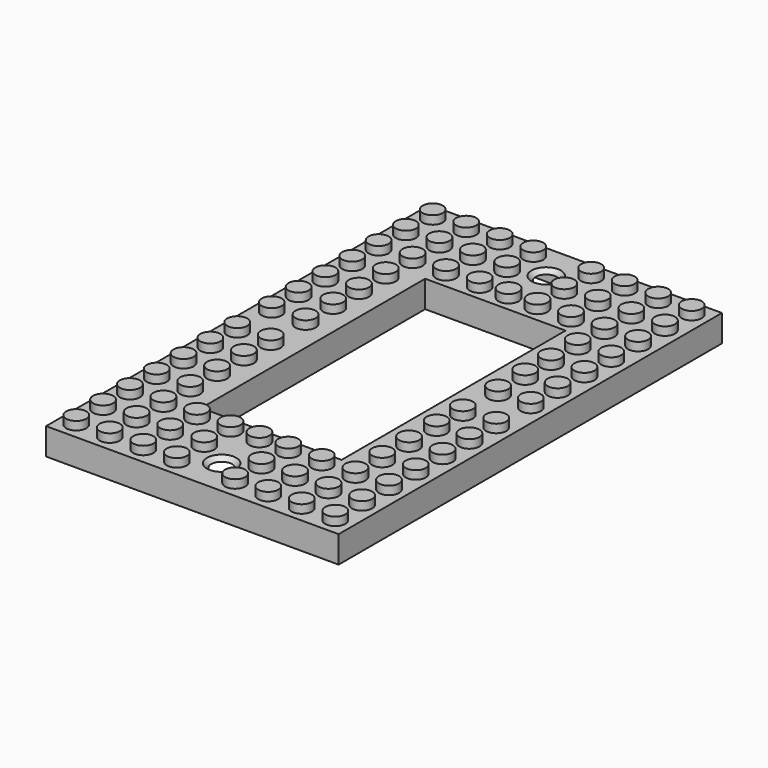
from build123d import *

# Parameters (mm, degrees)
F0_W           = 69.8
F0_H           = 114.3
F0_W_2         = 33.5
F0_H_2         = 66.8
F1_DEPTH       = 6.4
F2_T           = -1
F3_R           = 2.4
F4_DEPTH       = 2
F5_DEPTH       = 2
F6_D           = 4
F6_CSINK_D     = 7
F6_CSINK_ANGLE = 90
F7_D           = 4
F7_CSINK_D     = 7
F7_CSINK_ANGLE = 90


# Not quite as in the source:
# - a feature names something its author has since deleted; it is built from what else it names


with BuildPart() as f1:
    # F0 (on Top) → F1 (new body)
    with BuildSketch(Plane.XY):
        with Locations((0, 8.7452211694)):
            Rectangle(F0_W, F0_H)
        with Locations((-0.15, 8.7452211694)):
            Rectangle(F0_W_2, F0_H_2, mode=Mode.SUBTRACT)
    extrude(amount=F1_DEPTH)

    # F2
    f2_openings = [f1.faces().sort_by_distance(p)[0] for p in [
        (0, 64.555948, 0),
    ]]
    offset(amount=F2_T, openings=f2_openings, kind=Kind.INTERSECTION)

    # F3 (on face) → F4 (join)
    with BuildSketch(Plane.XY.offset(6.4)):
        with Locations((30.9, -44.4047788306)):
            Circle(F3_R)
        with Locations((22.9, -44.4047788306)):
            Circle(F3_R)
        with Locations((14.9, -44.4047788306)):
            Circle(F3_R)
        with Locations((6.9, -44.2756973207)):
            Circle(F3_R)
        with Locations((-6.9, -44.4047788306)):
            Circle(F3_R)
        with Locations((-14.9, -44.4047788306)):
            Circle(F3_R)
        with Locations((-22.9, -44.4047788306)):
            Circle(F3_R)
        with Locations((-30.9, -44.4047788306)):
            Circle(F3_R)
        with Locations((-30.9, -36.4047788306)):
            Circle(F3_R)
        with Locations((-22.9, -36.4047788306)):
            Circle(F3_R)
        with Locations((-14.9, -36.4047788306)):
            Circle(F3_R)
        with Locations((-6.9, -36.2545885146)):
            Circle(F3_R)
        with Locations((6.9, -36.4047788306)):
            Circle(F3_R)
        with Locations((14.9, -36.4047788306)):
            Circle(F3_R)
        with Locations((22.9, -36.4047788306)):
            Circle(F3_R)
        with Locations((30.9, -36.4047788306)):
            Circle(F3_R)
        with Locations((30.9, -28.4047788306)):
            Circle(F3_R)
        with Locations((22.9, -28.4047788306)):
            Circle(F3_R)
        with Locations((14.9, -28.4047788306)):
            Circle(F3_R)
        with Locations((6.9, -28.4047788306)):
            Circle(F3_R)
        with Locations((0, -28.4047788306)):
            Circle(F3_R)
        with Locations((-6.9, -28.4047788306)):
            Circle(F3_R)
        with Locations((-14.9, -28.4047788306)):
            Circle(F3_R)
        with Locations((-22.9, -28.4047788306)):
            Circle(F3_R)
        with Locations((-30.9, -28.4047788306)):
            Circle(F3_R)
        with Locations((-30.9, -20.4047788306)):
            Circle(F3_R)
        with Locations((-22.9, -20.4047788306)):
            Circle(F3_R)
        with Locations((22.9, -20.4047788306)):
            Circle(F3_R)
        with Locations((30.9, -20.4047788306)):
            Circle(F3_R)
        with Locations((-30.9, -12.4047788306)):
            Circle(F3_R)
        with Locations((-30.9, -4.4047788306)):
            Circle(F3_R)
        with Locations((-30.9, 3.5952211694)):
            Circle(F3_R)
        with Locations((-30.9, 13.8952211694)):
            Circle(F3_R)
        with Locations((-30.9, 29.8952211694)):
            Circle(F3_R)
        with Locations((-30.9, 21.8952211694)):
            Circle(F3_R)
        with Locations((-30.9, 37.8952211694)):
            Circle(F3_R)
        with Locations((-22.9, 37.8952211694)):
            Circle(F3_R)
        with Locations((-22.9, 29.8952211694)):
            Circle(F3_R)
        with Locations((-22.9, 22.2151018679)):
            Circle(F3_R)
        with Locations((-22.9, 13.9829078689)):
            Circle(F3_R)
        with Locations((-22.9, 3.5952211694)):
            Circle(F3_R)
        with Locations((-22.9, -4.4047788306)):
            Circle(F3_R)
        with Locations((-22.9, -12.4047788306)):
            Circle(F3_R)
        with Locations((22.9, -12.4047788306)):
            Circle(F3_R)
        with Locations((22.9, -4.1701360606)):
            Circle(F3_R)
        with Locations((22.9, 3.6398950033)):
            Circle(F3_R)
        with Locations((23.0275392532, 13.9829078689)):
            Circle(F3_R)
        with Locations((22.9, 22.2151018679)):
            Circle(F3_R)
        with Locations((22.9, 29.8952211694)):
            Circle(F3_R)
        with Locations((22.9, 37.8952211694)):
            Circle(F3_R)
        with Locations((30.9, 37.8952211694)):
            Circle(F3_R)
        with Locations((30.9, 29.8952211694)):
            Circle(F3_R)
        with Locations((30.9, 21.8952211694)):
            Circle(F3_R)
        with Locations((30.9, 13.8952211694)):
            Circle(F3_R)
        with Locations((30.9, 3.5952211694)):
            Circle(F3_R)
        with Locations((30.9, -4.4047788306)):
            Circle(F3_R)
        with Locations((30.9, -12.4047788306)):
            Circle(F3_R)
        with Locations((-30.9, 61.8952211694)):
            Circle(F3_R)
        with Locations((-30.9, 53.8952211694)):
            Circle(F3_R)
        with Locations((-31.0094300658, 45.8952211694)):
            Circle(F3_R)
        with Locations((-22.9, 45.8952211694)):
            Circle(F3_R)
        with Locations((-22.9, 53.8952211694)):
            Circle(F3_R)
        with Locations((-22.9, 61.8952211694)):
            Circle(F3_R)
        with Locations((-14.9, 61.8952211694)):
            Circle(F3_R)
        with Locations((-14.9, 53.8952211694)):
            Circle(F3_R)
        with Locations((-14.9, 45.8562783897)):
            Circle(F3_R)
        with Locations((-6.9, 45.8952211694)):
            Circle(F3_R)
        with Locations((-6.9, 54.08847332)):
            Circle(F3_R)
        with Locations((-6.9, 61.8952211694)):
            Circle(F3_R)
        with Locations((6.9, 61.8952211694)):
            Circle(F3_R)
        with Locations((0, 45.8952211694)):
            Circle(F3_R)
        with Locations((6.9, 45.8952211694)):
            Circle(F3_R)
        with Locations((6.9, 53.8773909211)):
            Circle(F3_R)
        with Locations((14.9, 61.8952211694)):
            Circle(F3_R)
        with Locations((14.9, 53.8952211694)):
            Circle(F3_R)
        with Locations((14.9, 45.8952211694)):
            Circle(F3_R)
        with Locations((22.9, 53.8952211694)):
            Circle(F3_R)
        with Locations((22.9, 61.8952211694)):
            Circle(F3_R)
        with Locations((30.9, 61.8952211694)):
            Circle(F3_R)
        with Locations((30.9, 53.8952211694)):
            Circle(F3_R)
        with Locations((30.9, 45.8952211694)):
            Circle(F3_R)
    extrude(amount=F4_DEPTH)

    # F3 (on face) → F5 (join)
    with BuildSketch(Plane.XY.offset(6.4)):
        with Locations((22.9, 45.8952211694)):
            Circle(F3_R)
    extrude(amount=F5_DEPTH)

    # F6 (through all)
    with Locations(Plane.XY.offset(6.4)):
        with Locations((0, 57.1199804544)):
            CounterSinkHole(F6_D / 2, F6_CSINK_D / 2, counter_sink_angle=F6_CSINK_ANGLE)

    # F7 (through all)
    with Locations(Plane.XY.offset(6.4)):
        with Locations((0, -39.6666899323)):
            CounterSinkHole(F7_D / 2, F7_CSINK_D / 2, counter_sink_angle=F7_CSINK_ANGLE)


solid = f1.part
